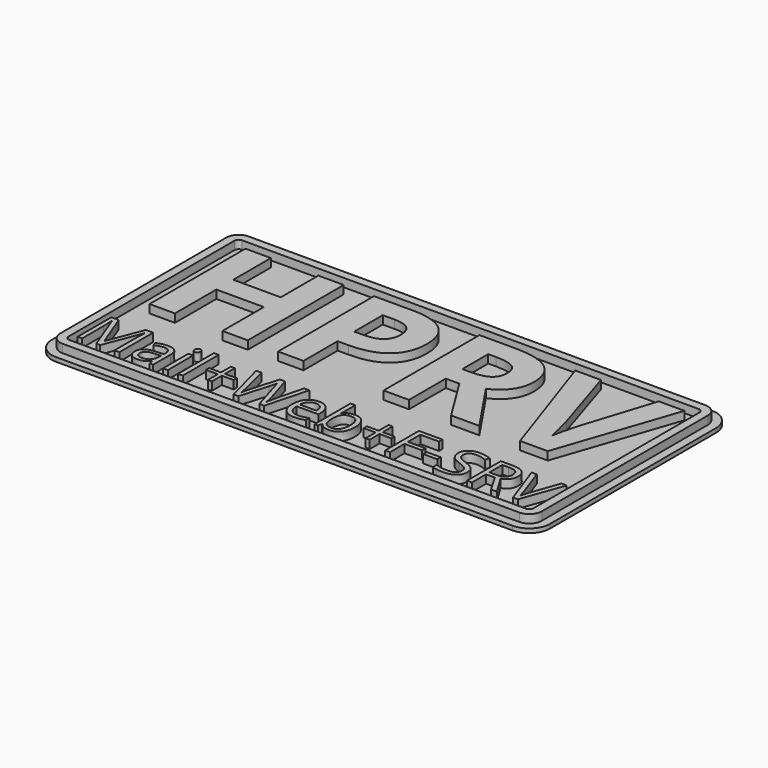
from build123d import *

# Parameters (mm, degrees)
F3_DEPTH       = 1
F4_TEXT_SIZE   = 40.4628845611
F4_TEXT_SIZE_2 = 14.2261739372
F5_DEPTH       = 2


# Not quite as in the source:
# - a feature names something its author has since deleted; it is built from what else it names
# - Text() gives the source's letters only with a copy of the font that has no kerning and outlines rounded to 1/6400 em; it was checked with that copy


with BuildPart() as f3:
    # F2 (on Top) → F3 (new body)
    with BuildSketch(Plane.XY):
        with BuildLine():
            Line((55, 30), (-55, 30))
            ThreePointArc((-55, 30), (-58.5355339059, 28.5355339059), (-60, 25))
            Line((-60, 25), (-60, -25))
            ThreePointArc((-60, -25), (-58.5355339059, -28.5355339059), (-55, -30))
            Line((-55, -30), (55, -30))
            ThreePointArc((55, -30), (58.5355339059, -28.5355339059), (60, -25))
            Line((60, -25), (60, 25))
            ThreePointArc((60, 25), (58.5355339059, 28.5355339059), (55, 30))
        make_face()
    extrude(amount=F3_DEPTH)

    # F4 (on face) → F5 (join)
    with BuildSketch(Plane.XY.offset(1)):
        with BuildLine():
            Line((55, 28), (-55, 28))
            ThreePointArc((-55, 28), (-57.1213203436, 27.1213203436), (-58, 25))
            Line((-58, 25), (-58, -25))
            ThreePointArc((-58, -25), (-57.1213203436, -27.1213203436), (-55, -28))
            Line((-55, -28), (55, -28))
            ThreePointArc((55, -28), (57.1213203436, -27.1213203436), (58, -25))
            Line((58, -25), (58, 25))
            ThreePointArc((58, 25), (57.1213203436, 27.1213203436), (55, 28))
        make_face()
        with BuildLine():
            ThreePointArc((-56, 25), (-55.7071067812, 25.7071067812), (-55, 26))
            Line((-55, 26), (55, 26))
            ThreePointArc((55, 26), (55.7071067812, 25.7071067812), (56, 25))
            Line((56, 25), (56, -25))
            ThreePointArc((56, -25), (55.7071067812, -25.7071067812), (55, -26))
            Line((55, -26), (-55, -26))
            ThreePointArc((-55, -26), (-55.7071067812, -25.7071067812), (-56, -25))
            Line((-56, -25), (-56, 25))
        make_face(mode=Mode.SUBTRACT)
        with Locations((-56, -5.1445211919)):
            Text('HPRV', F4_TEXT_SIZE, font='Open Sans', font_style=FontStyle.BOLD, text_align=(TextAlign.LEFT, TextAlign.BOTTOM))
        with Locations((-56, -23.9887556921)):
            Text('Mail+Web+F-SRV', F4_TEXT_SIZE_2, font='Open Sans', text_align=(TextAlign.LEFT, TextAlign.BOTTOM))
    extrude(amount=F5_DEPTH)


solid = f3.part
